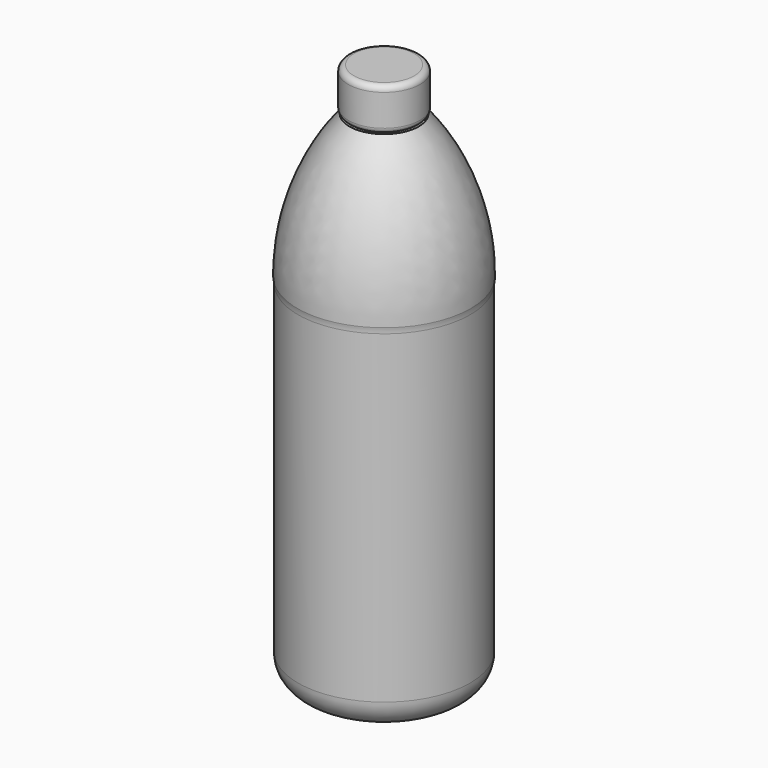
from build123d import *

# Parameters (mm, degrees)
F0_W = 76.2
F0_H = 317.5
F2_W = 31.75
F2_H = 38.1
F7_R = 5.08


# Not quite as in the source:
# - a fillet or chamfer that OpenCascade refuses, or shapes differently, is made with other operations: its cross-section is extruded or revolved along the edge and cut away or added


with BuildPart() as f1:
    # F0 (on Front) → F1 (revolve)
    with BuildSketch(Plane.XZ):
        with Locations((38.1, -158.75)):
            Rectangle(F0_W, F0_H)
    revolve(axis=Axis((0, 0, -158.75), (0, 0, -1)))

    # F4 (on Front) → F5 (revolve)
    with BuildSketch(Plane.XZ):
        with BuildLine():
            Line((30.7155977935, 126.9357353449), (0, 126.9357353449))
            Line((0, 126.9357353449), (0, 0))
            Line((0, 0), (76.7049640417, 0))
            ThreePointArc((76.7049640417, 0), (65.0449125042, 67.5744537485), (30.7155977935, 126.9357353449))
        make_face()
    revolve(axis=Axis((0, 0, 63.4678676724), (0, 0, -1)))

    # F6: fillet of radius 25.4 on 3 edges, made by hand

    # F6_s1 → F6_t2 (revolve)
    with BuildSketch(Plane.XZ):
        with BuildLine():
            ThreePointArc((76.7049640417, 0), (76.3265562958, -2.5071632184), (76.2, -5.0395619488))
            Line((76.2, -5.0395619488), (76.2, 0))
            Line((76.2, 0), (76.7049640417, 0))
        make_face()
    revolve(axis=Axis((0, 0, 0), (0, 0, -1)))

    # F6_s3 → F6_t4 (revolve, cut)
    with BuildSketch(Plane.XZ):
        with BuildLine():
            ThreePointArc((76.2, -292.1), (68.7605122421, -310.0605122421), (50.8, -317.5))
            Line((50.8, -317.5), (76.2, -317.5))
            Line((76.2, -317.5), (76.2, -292.1))
        make_face()
    revolve(axis=Axis((0, 0, -317.5), (0, 0, -1)), mode=Mode.SUBTRACT)


with BuildPart() as f3:
    # F2 (on Front) → F3 (revolve)
    with BuildSketch(Plane.XZ):
        with Locations((15.875, 146.05)):
            Rectangle(F2_W, F2_H)
    revolve(axis=Axis((0, 0, 146.05), (0, 0, -1)))

    # F7
    f7_edges = [f3.edges().sort_by_distance(p)[0] for p in [
        (-31.75, 0, 165.1),
        (-31.75, 0, 127),
        (31.75, 0, 146.05),
    ]]
    fillet(f7_edges, radius=F7_R)


solid = Compound([f1.part, f3.part])
